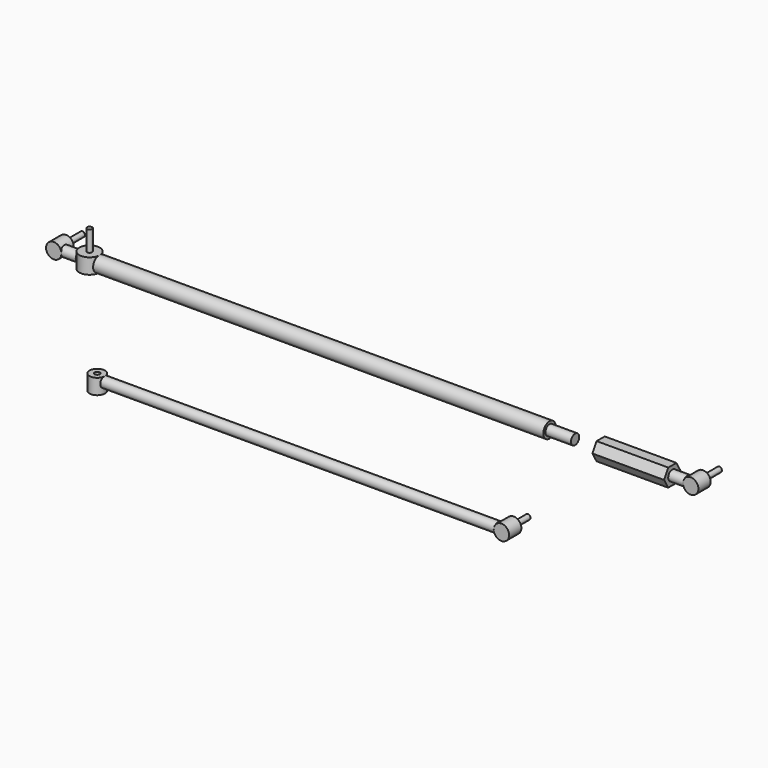
from build123d import *

# Parameters (mm, degrees)
F0_R      = 10
F1_DEPTH  = 140
F3_R      = 10
F4_DEPTH  = 70
F7_DEPTH  = 30
F9_DEPTH  = 60
F13_R     = 20
F14_DEPTH = 30
F15_R     = 5
F16_DEPTH = 55
F17_W     = 30
F17_H     = 10
F19_R     = 15
F20_DEPTH = 30
F21_R     = 5
F22_DEPTH = 60
F23_W     = 770
F23_H     = 10
F25_R     = 15
F26_DEPTH = 30
F27_R     = 5
F28_DEPTH = 55
F30_R     = 15
F30_R_2   = 5
F31_DEPTH = 30


with BuildPart() as f1:
    # F0 (on Right) → F1 (new body)
    with BuildSketch(Plane.YZ):
        Polygon((19.9997544387, -0.0991079843), (10.0857072515, 17.2707414212), (-9.9140471872, 17.3698494055), (-19.9997544387, 0.0991079843), (-10.0857072515, -17.2707414212), (9.9140471872, -17.3698494055), align=None)
        Circle(F0_R, mode=Mode.SUBTRACT)
    extrude(amount=F1_DEPTH)

    # F3 (on offset) → F4 (join)
    with BuildSketch(Plane.YZ.offset(100)):
        Circle(F3_R)
    extrude(amount=F4_DEPTH)

    # F6 (on offset) → F7 (join)
    with BuildSketch(Plane.XZ.offset(10)):
        with BuildLine():
            ThreePointArc((169, 0), (184, -15), (199, 0))
            ThreePointArc((199, 0), (184, 15), (169, 0))
        make_face()
    extrude(amount=-F7_DEPTH)

    # F8 (on Front) → F9 (join)
    with BuildSketch(Plane.XZ):
        with BuildLine():
            ThreePointArc((179, 0), (184, -5), (189, 0))
            ThreePointArc((189, 0), (184, 5), (179, 0))
        make_face()
    extrude(amount=-F9_DEPTH)


with BuildPart() as f11:
    # F10 (on Front) → F11 (revolve)
    with BuildSketch(Plane.XZ):
        Polygon((-980, 0), (-50, 0), (-50, 10), (-100, 10), (-100, 15), (-980, 15), align=None)
    revolve(axis=Axis((-515, 0, 0), (-1, 0, 0)))

    # F13 (on offset) → F14 (join)
    with BuildSketch(Plane.XY.offset(15)):
        with Locations((-999, 0)):
            Circle(F13_R)
    extrude(amount=-F14_DEPTH)

    # F15 (on Top) → F16 (join)
    with BuildSketch(Plane.XY):
        with Locations((-999, 0)):
            Circle(F15_R)
    extrude(amount=F16_DEPTH)

    # F17 (on Top) → F18 (revolve)
    with BuildSketch(Plane.XY):
        with Locations((-1033, 5)):
            Rectangle(F17_W, F17_H)
    revolve(axis=Axis((-1033, 0, 0), (-1, 0, 0)))

    # F19 (on offset) → F20 (join)
    with BuildSketch(Plane.XZ.offset(10)):
        with Locations((-1061, 0)):
            Circle(F19_R)
    extrude(amount=-F20_DEPTH)

    # F21 (on Front) → F22 (join)
    with BuildSketch(Plane.XZ):
        with Locations((-1061, 0)):
            Circle(F21_R)
    extrude(amount=-F22_DEPTH)


with BuildPart() as f24:
    # F23 (on Front) → F24 (revolve)
    with BuildSketch(Plane.XZ):
        with Locations((-585, -195)):
            Rectangle(F23_W, F23_H)
    revolve(axis=Axis((-585, 0, -200), (-1, 0, 0)))

    # F25 (on offset) → F26 (join)
    with BuildSketch(Plane.XZ.offset(10)):
        with Locations((-186, -200)):
            Circle(F25_R)
    extrude(amount=-F26_DEPTH)

    # F27 (on Front) → F28 (join)
    with BuildSketch(Plane.XZ):
        with Locations((-186, -200)):
            Circle(F27_R)
    extrude(amount=-F28_DEPTH)

    # F30 (on offset) → F31 (join)
    with BuildSketch(Plane.XY.offset(-190)):
        with Locations((-984, 0)):
            Circle(F30_R)
        with Locations((-984, 0)):
            Circle(F30_R_2, mode=Mode.SUBTRACT)
    extrude(amount=-F31_DEPTH)


solid = Compound([f1.part, f11.part, f24.part])
